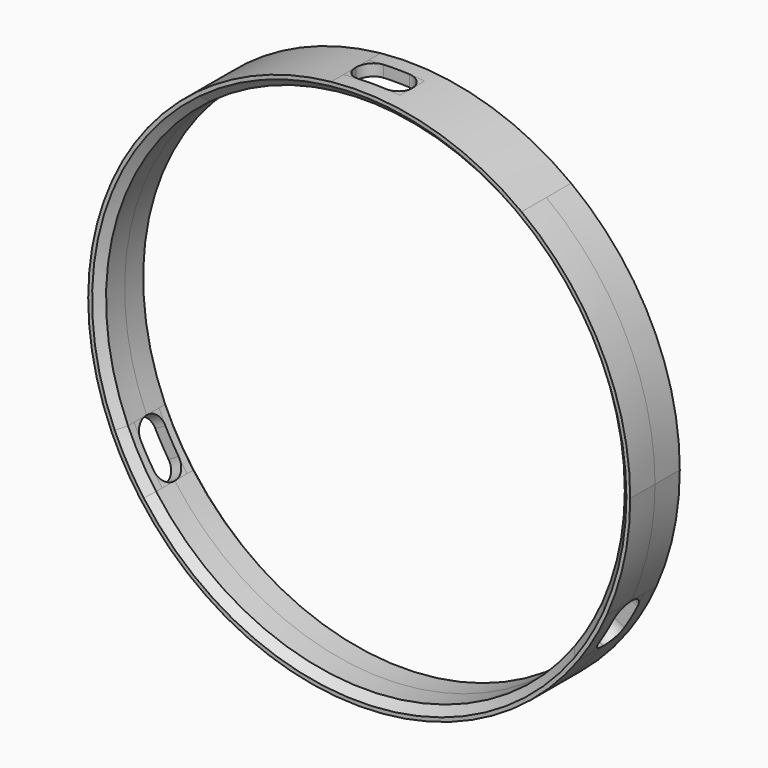
from build123d import *

# Parameters (mm, degrees)
F1_DEPTH      = 4
F1_DEPTH_BACK = 4
F2_SIZE       = 1
F4_DEPTH      = 2
F4_DEPTH_BACK = 2
F5_T4_DEPTH   = 11.2085158977
F5_S5_R       = 33.5
F5_T6_DEPTH   = 8
F5_S7_R       = 35
F5_T8_DEPTH   = 8
F5_T12_DEPTH  = 11.2085158977
F5_S13_R      = 35
F5_T14_DEPTH  = 8
F5_S15_R      = 33.5
F5_T16_DEPTH  = 8
F5_T20_DEPTH  = 11.2085158977
F5_S21_R      = 33.5
F5_T22_DEPTH  = 8
F5_S23_R      = 35
F5_T24_DEPTH  = 8
F5_T28_DEPTH  = 11.2085158977
F5_S29_R      = 33.5
F5_T30_DEPTH  = 8
F5_S31_R      = 35
F5_T32_DEPTH  = 8
F5_T36_DEPTH  = 11.2085158977
F5_S37_R      = 33.5
F5_T38_DEPTH  = 8
F5_S39_R      = 35
F5_T40_DEPTH  = 8
F5_T44_DEPTH  = 11.2085158977
F5_S45_R      = 33.5
F5_T46_DEPTH  = 8
F5_S47_R      = 35
F5_T48_DEPTH  = 8
F5_T52_DEPTH  = 11.2085158977
F5_S53_R      = 33.5
F5_T54_DEPTH  = 8
F5_S55_R      = 35
F5_T56_DEPTH  = 8
F5_T60_DEPTH  = 11.2085158977
F5_S61_R      = 33.5
F5_T62_DEPTH  = 8
F5_S63_R      = 35
F5_T64_DEPTH  = 8
F5_T68_DEPTH  = 11.2085158977
F5_S69_R      = 33.5
F5_T70_DEPTH  = 7
F5_S71_R      = 35
F5_T72_DEPTH  = 7
F5_T76_DEPTH  = 11.2085158977
F5_S77_R      = 33.5
F5_T78_DEPTH  = 7
F5_S79_R      = 35
F5_T80_DEPTH  = 7
F5_T84_DEPTH  = 11.2085158977
F5_S85_R      = 33.5
F5_T86_DEPTH  = 7
F5_S87_R      = 35
F5_T88_DEPTH  = 7
F5_T92_DEPTH  = 11.2085158977
F5_S93_R      = 33.5
F5_T94_DEPTH  = 7
F5_S95_R      = 35
F5_T96_DEPTH  = 7


# Not quite as in the source:
# - a fillet or chamfer that OpenCascade refuses, or shapes differently, is made with other operations: its cross-section is extruded or revolved along the edge and cut away or added


with BuildPart() as f1:
    # F0 (on Front) → F1 (new body, two sides)
    with BuildSketch(Plane.XZ) as f1_sk:
        with BuildLine():
            ThreePointArc((3.6332620451, 33.3023934112), (12.2794013905, 31.1683541672), (20.057750608, 26.8316350703))
            Line((20.057750608, 26.8316350703), (20.9639415908, 28.0270075637))
            ThreePointArc((20.9639415908, 28.0270075637), (12.7577794854, 32.5920091833), (3.6332620451, 34.8109093089))
            Line((3.6332620451, 34.8109093089), (3.6332620451, 33.3023934112))
        make_face()
        with BuildLine():
            ThreePointArc((-3.6332620451, 33.3023934112), (0, 33.5), (3.6332620451, 33.3023934112))
            Line((3.6332620451, 33.3023934112), (3.6332620451, 34.8109093089))
            ThreePointArc((3.6332620451, 34.8109093089), (0, 35), (-3.6332620451, 34.8109093089))
            Line((-3.6332620451, 34.8109093089), (-3.6332620451, 33.3023934112))
        make_face()
        with BuildLine():
            ThreePointArc((-20.057750608, 26.8316350703), (-12.2794013905, 31.1683541672), (-3.6332620451, 33.3023934112))
            Line((-3.6332620451, 33.3023934112), (-3.6332620451, 34.8109093089))
            ThreePointArc((-3.6332620451, 34.8109093089), (-12.7577794854, 32.5920091833), (-20.9639415908, 28.0270075637))
            Line((-20.9639415908, 28.0270075637), (-20.057750608, 26.8316350703))
        make_face()
        with BuildLine():
            ThreePointArc((-30.6573497234, -13.504699476), (-32.4000049624, 8.5140870583), (-20.057750608, 26.8316350703))
            Line((-20.057750608, 26.8316350703), (-20.9639415908, 28.0270075637))
            ThreePointArc((-20.9639415908, 28.0270075637), (-33.8727203235, 8.8112892295), (-31.9637628129, -14.2589574248))
            Line((-31.9637628129, -14.2589574248), (-30.6573497234, -13.504699476))
        make_face()
        with BuildLine():
            Line((-28.3305007678, -20.5519518841), (-27.0240876784, -19.7976939352))
            ThreePointArc((-27.0240876784, -19.7976939352), (-29.0118510268, -16.75), (-30.6573497234, -13.504699476))
            Line((-30.6573497234, -13.504699476), (-31.9637628129, -14.2589574248))
            ThreePointArc((-31.9637628129, -14.2589574248), (-30.3108891325, -17.5), (-28.3305007678, -20.5519518841))
        make_face()
        with BuildLine():
            Line((28.3305007678, -20.5519518841), (27.0240876784, -19.7976939352))
            ThreePointArc((27.0240876784, -19.7976939352), (0, -33.5), (-27.0240876784, -19.7976939352))
            Line((-27.0240876784, -19.7976939352), (-28.3305007678, -20.5519518841))
            ThreePointArc((-28.3305007678, -20.5519518841), (0, -35), (28.3305007678, -20.5519518841))
        make_face()
        with BuildLine():
            Line((31.9637628129, -14.2589574248), (30.6573497234, -13.504699476))
            ThreePointArc((30.6573497234, -13.504699476), (29.0118510268, -16.75), (27.0240876784, -19.7976939352))
            Line((27.0240876784, -19.7976939352), (28.3305007678, -20.5519518841))
            ThreePointArc((28.3305007678, -20.5519518841), (30.3108891325, -17.5), (31.9637628129, -14.2589574248))
        make_face()
        with BuildLine():
            ThreePointArc((20.057750608, 26.8316350703), (29.9514995064, 15.00525499), (33.5, 0))
            ThreePointArc((33.5, 0), (32.7816352226, -6.9003182631), (30.6573497234, -13.504699476))
            Line((30.6573497234, -13.504699476), (31.9637628129, -14.2589574248))
            ThreePointArc((31.9637628129, -14.2589574248), (34.2325261882, -7.2893175795), (35, 0))
            ThreePointArc((35, 0), (31.2948714303, 15.6726201434), (20.9639415908, 28.0270075637))
            Line((20.9639415908, 28.0270075637), (20.057750608, 26.8316350703))
        make_face()
        with BuildLine():
            Line((28.3305007678, -20.5519518841), (27.0240876784, -19.7976939352))
            ThreePointArc((27.0240876784, -19.7976939352), (0, -33.5), (-27.0240876784, -19.7976939352))
            Line((-27.0240876784, -19.7976939352), (-28.3305007678, -20.5519518841))
            ThreePointArc((-28.3305007678, -20.5519518841), (0, -35), (28.3305007678, -20.5519518841))
        make_face()
        with BuildLine():
            ThreePointArc((20.057750608, 26.8316350703), (29.9514995064, 15.00525499), (33.5, 0))
            ThreePointArc((33.5, 0), (32.7816352226, -6.9003182631), (30.6573497234, -13.504699476))
            Line((30.6573497234, -13.504699476), (31.9637628129, -14.2589574248))
            ThreePointArc((31.9637628129, -14.2589574248), (34.2325261882, -7.2893175795), (35, 0))
            ThreePointArc((35, 0), (31.2948714303, 15.6726201434), (20.9639415908, 28.0270075637))
            Line((20.9639415908, 28.0270075637), (20.057750608, 26.8316350703))
        make_face()
        with BuildLine():
            ThreePointArc((-30.6573497234, -13.504699476), (-32.4000049624, 8.5140870583), (-20.057750608, 26.8316350703))
            Line((-20.057750608, 26.8316350703), (-20.9639415908, 28.0270075637))
            ThreePointArc((-20.9639415908, 28.0270075637), (-33.8727203235, 8.8112892295), (-31.9637628129, -14.2589574248))
            Line((-31.9637628129, -14.2589574248), (-30.6573497234, -13.504699476))
        make_face()
        with BuildLine():
            Line((28.3305007678, -20.5519518841), (27.0240876784, -19.7976939352))
            ThreePointArc((27.0240876784, -19.7976939352), (0, -33.5), (-27.0240876784, -19.7976939352))
            Line((-27.0240876784, -19.7976939352), (-28.3305007678, -20.5519518841))
            ThreePointArc((-28.3305007678, -20.5519518841), (0, -35), (28.3305007678, -20.5519518841))
        make_face()
    extrude(amount=F1_DEPTH)
    extrude(f1_sk.sketch, amount=-F1_DEPTH_BACK)

    # F2
    f2_edges = [f1.edges().sort_by_distance(p)[0] for p in [
        (-30.65735, -4, 13.504699),
        (-30.65735, 4, 13.504699),
    ]]
    chamfer(f2_edges, length=F2_SIZE)

    # F0 (on Front) → F4 (cut, two sides)
    with BuildSketch(Plane.XZ) as f4_sk:
        with BuildLine():
            ThreePointArc((-3.6332620451, 34.8109093089), (0, 35), (3.6332620451, 34.8109093089))
            Line((3.6332620451, 34.8109093089), (3.6332620451, 36.968215256))
            Line((3.6332620451, 36.968215256), (-3.6332620451, 36.968215256))
            Line((-3.6332620451, 36.968215256), (-3.6332620451, 34.8109093089))
        make_face()
        with BuildLine():
            ThreePointArc((-3.6332620451, 33.3023934112), (0, 33.5), (3.6332620451, 33.3023934112))
            Line((3.6332620451, 33.3023934112), (3.6332620451, 34.8109093089))
            ThreePointArc((3.6332620451, 34.8109093089), (0, 35), (-3.6332620451, 34.8109093089))
            Line((-3.6332620451, 34.8109093089), (-3.6332620451, 33.3023934112))
        make_face()
        with BuildLine():
            Line((3.6332620451, 31.6989157826), (3.6332620451, 33.3023934112))
            ThreePointArc((3.6332620451, 33.3023934112), (0, 33.5), (-3.6332620451, 33.3023934112))
            Line((-3.6332620451, 33.3023934112), (-3.6332620451, 31.6989157826))
            Line((-3.6332620451, 31.6989157826), (3.6332620451, 31.6989157826))
        make_face()
        with BuildLine():
            ThreePointArc((27.0240876784, -19.7976939352), (29.0118510268, -16.75), (30.6573497234, -13.504699476))
            Line((30.6573497234, -13.504699476), (7.2665240901, 0))
            Line((7.2665240901, 0), (3.3491878185, -6.1289841281))
            Line((3.3491878185, -6.1289841281), (27.0240876784, -19.7976939352))
        make_face()
        with BuildLine():
            Line((31.9637628129, -14.2589574248), (30.6573497234, -13.504699476))
            ThreePointArc((30.6573497234, -13.504699476), (29.0118510268, -16.75), (27.0240876784, -19.7976939352))
            Line((27.0240876784, -19.7976939352), (28.3305007678, -20.5519518841))
            ThreePointArc((28.3305007678, -20.5519518841), (30.3108891325, -17.5), (31.9637628129, -14.2589574248))
        make_face()
        with BuildLine():
            Line((33.8320445668, -15.3376103984), (31.9637628129, -14.2589574248))
            ThreePointArc((31.9637628129, -14.2589574248), (30.3108891325, -17.5), (28.3305007678, -20.5519518841))
            Line((28.3305007678, -20.5519518841), (30.1987825217, -21.6306048576))
            Line((30.1987825217, -21.6306048576), (33.8320445668, -15.3376103984))
        make_face()
        with BuildLine():
            ThreePointArc((-30.6573497234, -13.504699476), (-29.0118510268, -16.75), (-27.0240876784, -19.7976939352))
            Line((-27.0240876784, -19.7976939352), (-3.2841431884, -6.0914305934))
            Line((-3.2841431884, -6.0914305934), (-6.8559292529, 0.2370570398))
            Line((-6.8559292529, 0.2370570398), (-30.6573497234, -13.504699476))
        make_face()
        with BuildLine():
            Line((-30.1987825217, -21.6306048576), (-28.3305007678, -20.5519518841))
            ThreePointArc((-28.3305007678, -20.5519518841), (-30.3108891325, -17.5), (-31.9637628129, -14.2589574248))
            Line((-31.9637628129, -14.2589574248), (-33.8320445668, -15.3376103984))
            Line((-33.8320445668, -15.3376103984), (-30.1987825217, -21.6306048576))
        make_face()
        with BuildLine():
            Line((-28.3305007678, -20.5519518841), (-27.0240876784, -19.7976939352))
            ThreePointArc((-27.0240876784, -19.7976939352), (-29.0118510268, -16.75), (-30.6573497234, -13.504699476))
            Line((-30.6573497234, -13.504699476), (-31.9637628129, -14.2589574248))
            ThreePointArc((-31.9637628129, -14.2589574248), (-30.3108891325, -17.5), (-28.3305007678, -20.5519518841))
        make_face()
    extrude(amount=-F4_DEPTH, mode=Mode.SUBTRACT)
    extrude(f4_sk.sketch, amount=F4_DEPTH_BACK, mode=Mode.SUBTRACT)

    # F5: fillet of radius 1.94 on 12 edges, made by hand


with BuildPart() as f5_tool2:
    # F5_s3 → F5_t4 (new body)
    with BuildSketch(Plane(origin=(24.6404954925, 0, -14.2261967056), x_dir=(0, 1, 0), z_dir=(0.8660254038, 0, -0.5))):
        with BuildLine():
            ThreePointArc((0.06, -3.6332620451), (1.4317871555, -3.0650492006), (2, -1.6932620451))
            Line((2, -1.6932620451), (2, -3.6332620451))
            Line((2, -3.6332620451), (0.06, -3.6332620451))
        make_face()
    extrude(amount=F5_T4_DEPTH)

    # F5_s5 → F5_t6 (cut, symmetric)
    with BuildSketch(Plane.XZ.offset(-1)):
        Circle(F5_S5_R)
    extrude(amount=F5_T6_DEPTH, both=True, mode=Mode.SUBTRACT)

    # F5_s7 → F5_t8 (intersect, symmetric)
    with BuildSketch(Plane.XZ.offset(-1)):
        Circle(F5_S7_R)
    extrude(amount=F5_T8_DEPTH, both=True, mode=Mode.INTERSECT)


with BuildPart() as f1_1:
    add(f1.part)

    # F5_t1: union F5_tool2
    add(f5_tool2.part)


with BuildPart() as f5_tool10:
    # F5_s11 → F5_t12 (new body)
    with BuildSketch(Plane(origin=(34.3473549987, 0, -19.8304546544), x_dir=(0, 1, 0), z_dir=(-0.8660254038, 0, 0.5))):
        with BuildLine():
            ThreePointArc((0.06, -3.6332620451), (1.4317871555, -3.0650492006), (2, -1.6932620451))
            Line((2, -1.6932620451), (2, -3.6332620451))
            Line((2, -3.6332620451), (0.06, -3.6332620451))
        make_face()
    extrude(amount=F5_T12_DEPTH)

    # F5_s13 → F5_t14 (intersect, symmetric)
    with BuildSketch(Plane.XZ.offset(-1)):
        Circle(F5_S13_R)
    extrude(amount=F5_T14_DEPTH, both=True, mode=Mode.INTERSECT)

    # F5_s15 → F5_t16 (cut, symmetric)
    with BuildSketch(Plane.XZ.offset(-1)):
        Circle(F5_S15_R)
    extrude(amount=F5_T16_DEPTH, both=True, mode=Mode.SUBTRACT)


with BuildPart() as f1_2:
    add(f1_1.part)

    # F5_t9: union F5_tool10
    add(f5_tool10.part)


with BuildPart() as f5_tool18:
    # F5_s19 → F5_t20 (new body)
    with BuildSketch(Plane(origin=(34.3473549987, 0, -19.8304546544), x_dir=(0, 1, 0), z_dir=(-0.8660254038, 0, 0.5))):
        with BuildLine():
            ThreePointArc((-0.06, -3.6332620451), (-1.4317871555, -3.0650492006), (-2, -1.6932620451))
            Line((-2, -1.6932620451), (-2, -3.6332620451))
            Line((-2, -3.6332620451), (-0.06, -3.6332620451))
        make_face()
    extrude(amount=F5_T20_DEPTH)

    # F5_s21 → F5_t22 (cut, symmetric)
    with BuildSketch(Plane.XZ.offset(1)):
        Circle(F5_S21_R)
    extrude(amount=F5_T22_DEPTH, both=True, mode=Mode.SUBTRACT)

    # F5_s23 → F5_t24 (intersect, symmetric)
    with BuildSketch(Plane.XZ.offset(1)):
        Circle(F5_S23_R)
    extrude(amount=F5_T24_DEPTH, both=True, mode=Mode.INTERSECT)


with BuildPart() as f1_3:
    add(f1_2.part)

    # F5_t17: union F5_tool18
    add(f5_tool18.part)


with BuildPart() as f5_tool26:
    # F5_s27 → F5_t28 (new body)
    with BuildSketch(Plane(origin=(24.6404954925, 0, -14.2261967056), x_dir=(0, 1, 0), z_dir=(0.8660254038, 0, -0.5))):
        with BuildLine():
            ThreePointArc((-2, -1.6932620451), (-1.4317871555, -3.0650492006), (-0.06, -3.6332620451))
            Line((-0.06, -3.6332620451), (-2, -3.6332620451))
            Line((-2, -3.6332620451), (-2, -1.6932620451))
        make_face()
    extrude(amount=F5_T28_DEPTH)

    # F5_s29 → F5_t30 (cut, symmetric)
    with BuildSketch(Plane.XZ.offset(1)):
        Circle(F5_S29_R)
    extrude(amount=F5_T30_DEPTH, both=True, mode=Mode.SUBTRACT)

    # F5_s31 → F5_t32 (intersect, symmetric)
    with BuildSketch(Plane.XZ.offset(1)):
        Circle(F5_S31_R)
    extrude(amount=F5_T32_DEPTH, both=True, mode=Mode.INTERSECT)


with BuildPart() as f1_4:
    add(f1_3.part)

    # F5_t25: union F5_tool26
    add(f5_tool26.part)


with BuildPart() as f5_tool34:
    # F5_s35 → F5_t36 (new body)
    with BuildSketch(Plane(origin=(-34.3473549987, 0, -19.8304546544), x_dir=(0, 1, 0), z_dir=(0.8660254038, 0, 0.5))):
        with BuildLine():
            ThreePointArc((0.06, -3.6332620451), (1.4317871555, -3.0650492006), (2, -1.6932620451))
            Line((2, -1.6932620451), (2, -3.6332620451))
            Line((2, -3.6332620451), (0.06, -3.6332620451))
        make_face()
    extrude(amount=F5_T36_DEPTH)

    # F5_s37 → F5_t38 (cut, symmetric)
    with BuildSketch(Plane.XZ.offset(-1)):
        Circle(F5_S37_R)
    extrude(amount=F5_T38_DEPTH, both=True, mode=Mode.SUBTRACT)

    # F5_s39 → F5_t40 (intersect, symmetric)
    with BuildSketch(Plane.XZ.offset(-1)):
        Circle(F5_S39_R)
    extrude(amount=F5_T40_DEPTH, both=True, mode=Mode.INTERSECT)


with BuildPart() as f1_5:
    add(f1_4.part)

    # F5_t33: union F5_tool34
    add(f5_tool34.part)


with BuildPart() as f5_tool42:
    # F5_s43 → F5_t44 (new body)
    with BuildSketch(Plane(origin=(-24.6404954925, 0, -14.2261967056), x_dir=(0, 1, 0), z_dir=(-0.8660254038, 0, -0.5))):
        with BuildLine():
            ThreePointArc((0.06, -3.6332620451), (1.4317871555, -3.0650492006), (2, -1.6932620451))
            Line((2, -1.6932620451), (2, -3.6332620451))
            Line((2, -3.6332620451), (0.06, -3.6332620451))
        make_face()
    extrude(amount=F5_T44_DEPTH)

    # F5_s45 → F5_t46 (cut, symmetric)
    with BuildSketch(Plane.XZ.offset(-1)):
        Circle(F5_S45_R)
    extrude(amount=F5_T46_DEPTH, both=True, mode=Mode.SUBTRACT)

    # F5_s47 → F5_t48 (intersect, symmetric)
    with BuildSketch(Plane.XZ.offset(-1)):
        Circle(F5_S47_R)
    extrude(amount=F5_T48_DEPTH, both=True, mode=Mode.INTERSECT)


with BuildPart() as f1_6:
    add(f1_5.part)

    # F5_t41: union F5_tool42
    add(f5_tool42.part)


with BuildPart() as f5_tool50:
    # F5_s51 → F5_t52 (new body)
    with BuildSketch(Plane(origin=(-24.6404954925, 0, -14.2261967056), x_dir=(0, 1, 0), z_dir=(-0.8660254038, 0, -0.5))):
        with BuildLine():
            ThreePointArc((-2, -1.6932620451), (-1.4317871555, -3.0650492006), (-0.06, -3.6332620451))
            Line((-0.06, -3.6332620451), (-2, -3.6332620451))
            Line((-2, -3.6332620451), (-2, -1.6932620451))
        make_face()
    extrude(amount=F5_T52_DEPTH)

    # F5_s53 → F5_t54 (cut, symmetric)
    with BuildSketch(Plane.XZ.offset(1)):
        Circle(F5_S53_R)
    extrude(amount=F5_T54_DEPTH, both=True, mode=Mode.SUBTRACT)

    # F5_s55 → F5_t56 (intersect, symmetric)
    with BuildSketch(Plane.XZ.offset(1)):
        Circle(F5_S55_R)
    extrude(amount=F5_T56_DEPTH, both=True, mode=Mode.INTERSECT)


with BuildPart() as f1_7:
    add(f1_6.part)

    # F5_t49: union F5_tool50
    add(f5_tool50.part)


with BuildPart() as f5_tool58:
    # F5_s59 → F5_t60 (new body)
    with BuildSketch(Plane(origin=(-34.3473549987, 0, -19.8304546544), x_dir=(0, 1, 0), z_dir=(0.8660254038, 0, 0.5))):
        with BuildLine():
            ThreePointArc((-0.06, -3.6332620451), (-1.4317871555, -3.0650492006), (-2, -1.6932620451))
            Line((-2, -1.6932620451), (-2, -3.6332620451))
            Line((-2, -3.6332620451), (-0.06, -3.6332620451))
        make_face()
    extrude(amount=F5_T60_DEPTH)

    # F5_s61 → F5_t62 (cut, symmetric)
    with BuildSketch(Plane.XZ.offset(1)):
        Circle(F5_S61_R)
    extrude(amount=F5_T62_DEPTH, both=True, mode=Mode.SUBTRACT)

    # F5_s63 → F5_t64 (intersect, symmetric)
    with BuildSketch(Plane.XZ.offset(1)):
        Circle(F5_S63_R)
    extrude(amount=F5_T64_DEPTH, both=True, mode=Mode.INTERSECT)


with BuildPart() as f1_8:
    add(f1_7.part)

    # F5_t57: union F5_tool58
    add(f5_tool58.part)


with BuildPart() as f5_tool66:
    # F5_s67 → F5_t68 (new body)
    with BuildSketch(Plane.XY.offset(39.6609093089)):
        with BuildLine():
            ThreePointArc((-3.6332620451, 0.06), (-3.0650492006, 1.4317871555), (-1.6932620451, 2))
            Line((-1.6932620451, 2), (-3.6332620451, 2))
            Line((-3.6332620451, 2), (-3.6332620451, 0.06))
        make_face()
    extrude(amount=-F5_T68_DEPTH)

    # F5_s69 → F5_t70 (cut, symmetric)
    with BuildSketch(Plane.XZ.offset(-1)):
        Circle(F5_S69_R)
    extrude(amount=F5_T70_DEPTH, both=True, mode=Mode.SUBTRACT)

    # F5_s71 → F5_t72 (intersect, symmetric)
    with BuildSketch(Plane.XZ.offset(-1)):
        Circle(F5_S71_R)
    extrude(amount=F5_T72_DEPTH, both=True, mode=Mode.INTERSECT)


with BuildPart() as f1_9:
    add(f1_8.part)

    # F5_t65: union F5_tool66
    add(f5_tool66.part)


with BuildPart() as f5_tool74:
    # F5_s75 → F5_t76 (new body)
    with BuildSketch(Plane.XY.offset(28.4523934112)):
        with BuildLine():
            ThreePointArc((3.6332620451, 0.06), (3.0650492006, 1.4317871555), (1.6932620451, 2))
            Line((1.6932620451, 2), (3.6332620451, 2))
            Line((3.6332620451, 2), (3.6332620451, 0.06))
        make_face()
    extrude(amount=F5_T76_DEPTH)

    # F5_s77 → F5_t78 (cut, symmetric)
    with BuildSketch(Plane.XZ.offset(-1)):
        Circle(F5_S77_R)
    extrude(amount=F5_T78_DEPTH, both=True, mode=Mode.SUBTRACT)

    # F5_s79 → F5_t80 (intersect, symmetric)
    with BuildSketch(Plane.XZ.offset(-1)):
        Circle(F5_S79_R)
    extrude(amount=F5_T80_DEPTH, both=True, mode=Mode.INTERSECT)


with BuildPart() as f1_10:
    add(f1_9.part)

    # F5_t73: union F5_tool74
    add(f5_tool74.part)


with BuildPart() as f5_tool82:
    # F5_s83 → F5_t84 (new body)
    with BuildSketch(Plane.XY.offset(39.6609093089)):
        with BuildLine():
            ThreePointArc((-3.6332620451, -0.06), (-3.0650492006, -1.4317871555), (-1.6932620451, -2))
            Line((-1.6932620451, -2), (-3.6332620451, -2))
            Line((-3.6332620451, -2), (-3.6332620451, -0.06))
        make_face()
    extrude(amount=-F5_T84_DEPTH)

    # F5_s85 → F5_t86 (cut, symmetric)
    with BuildSketch(Plane.XZ.offset(1)):
        Circle(F5_S85_R)
    extrude(amount=F5_T86_DEPTH, both=True, mode=Mode.SUBTRACT)

    # F5_s87 → F5_t88 (intersect, symmetric)
    with BuildSketch(Plane.XZ.offset(1)):
        Circle(F5_S87_R)
    extrude(amount=F5_T88_DEPTH, both=True, mode=Mode.INTERSECT)


with BuildPart() as f1_11:
    add(f1_10.part)

    # F5_t81: union F5_tool82
    add(f5_tool82.part)


with BuildPart() as f5_tool90:
    # F5_s91 → F5_t92 (new body)
    with BuildSketch(Plane.XY.offset(28.4523934112)):
        with BuildLine():
            ThreePointArc((1.6932620451, -2), (3.0650492006, -1.4317871555), (3.6332620451, -0.06))
            Line((3.6332620451, -0.06), (3.6332620451, -2))
            Line((3.6332620451, -2), (1.6932620451, -2))
        make_face()
    extrude(amount=F5_T92_DEPTH)

    # F5_s93 → F5_t94 (cut, symmetric)
    with BuildSketch(Plane.XZ.offset(1)):
        Circle(F5_S93_R)
    extrude(amount=F5_T94_DEPTH, both=True, mode=Mode.SUBTRACT)

    # F5_s95 → F5_t96 (intersect, symmetric)
    with BuildSketch(Plane.XZ.offset(1)):
        Circle(F5_S95_R)
    extrude(amount=F5_T96_DEPTH, both=True, mode=Mode.INTERSECT)


with BuildPart() as f1_12:
    add(f1_11.part)

    # F5_t89: union F5_tool90
    add(f5_tool90.part)


solid = f1_12.part
